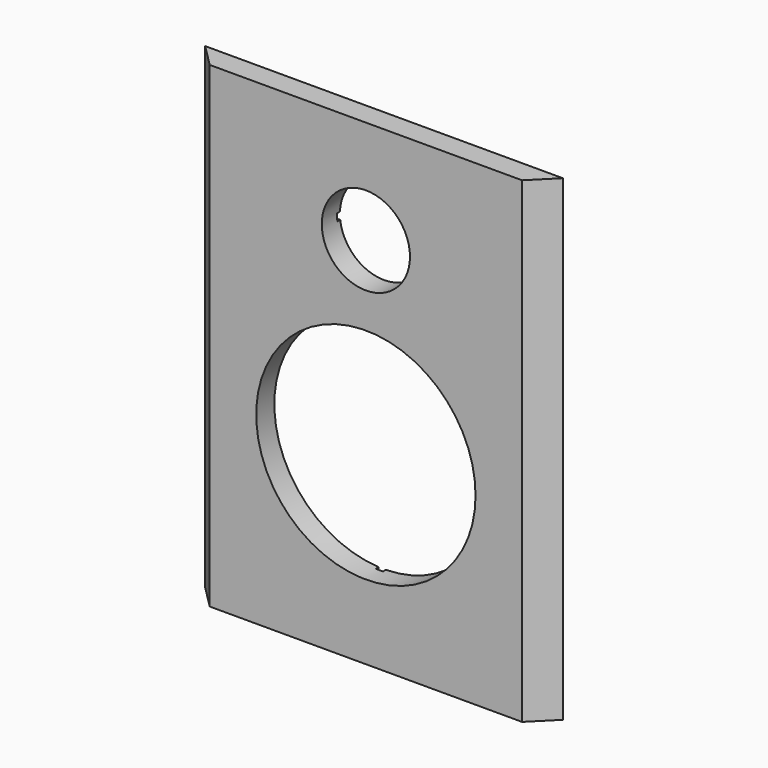
from build123d import *

# Parameters (mm, degrees)
F0_W     = 300
F0_H     = 400
F1_DEPTH = 19
F2_R     = 37
F2_R_2   = 92
F3_DEPTH = 19
F4_SIZE  = 18.99999
F6_DEPTH = 3
F7_W     = 6
F7_H     = 64.6666483516
F8_DEPTH = 3


# Not quite as in the source:
# - a fillet or chamfer is up to 0.001 mm smaller than in the source, because OpenCascade refuses the exact size


with BuildPart() as f1:
    # F0 (on Front) → F1 (new body)
    with BuildSketch(Plane.XZ):
        with Locations((-100.0432893634, -3.2491389651)):
            Rectangle(F0_W, F0_H)
    extrude(amount=F1_DEPTH)

    # F2 (on face) → F3 (cut)
    with BuildSketch(Plane.XZ.offset(19)):
        with Locations((-100.0432893634, 109.7508610349)):
            Circle(F2_R)
        with Locations((-100.0432893634, -48.7491389651)):
            Circle(F2_R_2)
    extrude(amount=-F3_DEPTH, mode=Mode.SUBTRACT)

    # F4 (size 19 in the source; OpenCascade refuses exactly that, so slightly less here)
    f4_edges = [f1.edges().sort_by_distance(p)[0] for p in [
        (-250.043289, -19, -3.249139),
        (49.956711, -19, -3.249139),
    ]]
    chamfer(f4_edges, length=F4_SIZE)

    # F5 (on face) → F6 (cut)
    with BuildSketch(Plane(origin=(0, 0, 0), x_dir=(-1, 0, 0), z_dir=(0, 1, 0))):
        Polygon((136.7686212203, 111.2508610349), (136.7686212203, 105.2508610349), (212.0432893634, 105.2508610349), (212.0432893634, -194.7491389651), (218.0432893634, -194.7491389651), (218.0432893634, 111.2508610349), align=None)
    extrude(amount=-F6_DEPTH, mode=Mode.SUBTRACT)

    # F7 (on face) → F8 (cut)
    with BuildSketch(Plane(origin=(0, 0, 0), x_dir=(-1, 0, 0), z_dir=(0, 1, 0))):
        with Locations((101.5432893634, -162.4158147893)):
            Rectangle(F7_W, F7_H)
    extrude(amount=-F8_DEPTH, mode=Mode.SUBTRACT)


solid = f1.part
